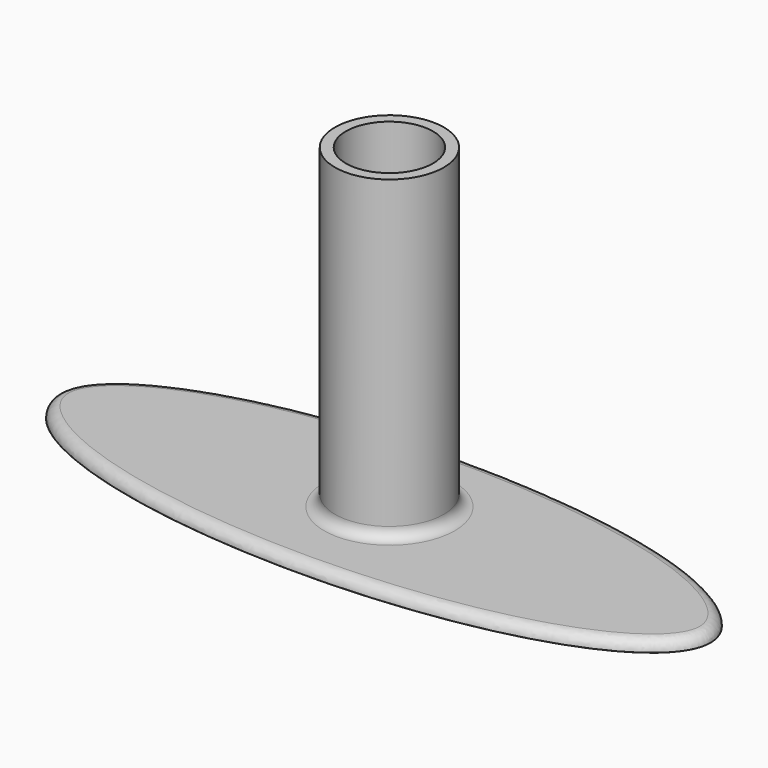
from build123d import *

# Parameters (mm, degrees)
F2_R     = 25
F2_R_2   = 19.999999553
F5_DEPTH = 5
F6_R     = 4.999


# Not quite as in the source:
# - a fillet or chamfer is up to 0.001 mm smaller than in the source, because OpenCascade refuses the exact size


with BuildPart() as f4:
    # F4: sweep along a path in F3
    with BuildLine(Plane.XZ) as f4_path:
        Line((0, 150.3136307001), (0, 0))
    # F2 (on offset) → F4 (sweep)
    with BuildSketch(Plane.XY.offset(150)):
        with Locations((0, 3.1161449583)):
            Circle(F2_R)
        with Locations((0, 3.1161449583)):
            Circle(F2_R_2, mode=Mode.SUBTRACT)
    sweep(path=f4_path.line)

    # F0 (on Top) → F5 (join)
    with BuildSketch(Plane.XY):
        with BuildLine():
            add(Edge.make_bspline(
                [(150, 0), (150, 86.6025403784), (-75, 43.3012701892), (-300, 0), (-75, -43.3012701892), (150, -86.6025403784), (150, 0)],
                knots=[0, 0, 0, 2.0943951024, 2.0943951024, 4.1887902048, 4.1887902048, 6.2831853072, 6.2831853072, 6.2831853072], degree=2, weights=[1, 0.5, 1, 0.5, 1, 0.5, 1]))
        make_face()
    extrude(amount=F5_DEPTH)

    # F6 (radius 5 in the source; OpenCascade refuses exactly that, so slightly less here)
    f6_edges = [f4.edges().sort_by_distance(p)[0] for p in [
        (-150, 0.000863, 5),
        (-25, 3.116145, 5),
    ]]
    fillet(f6_edges, radius=F6_R)


solid = f4.part
